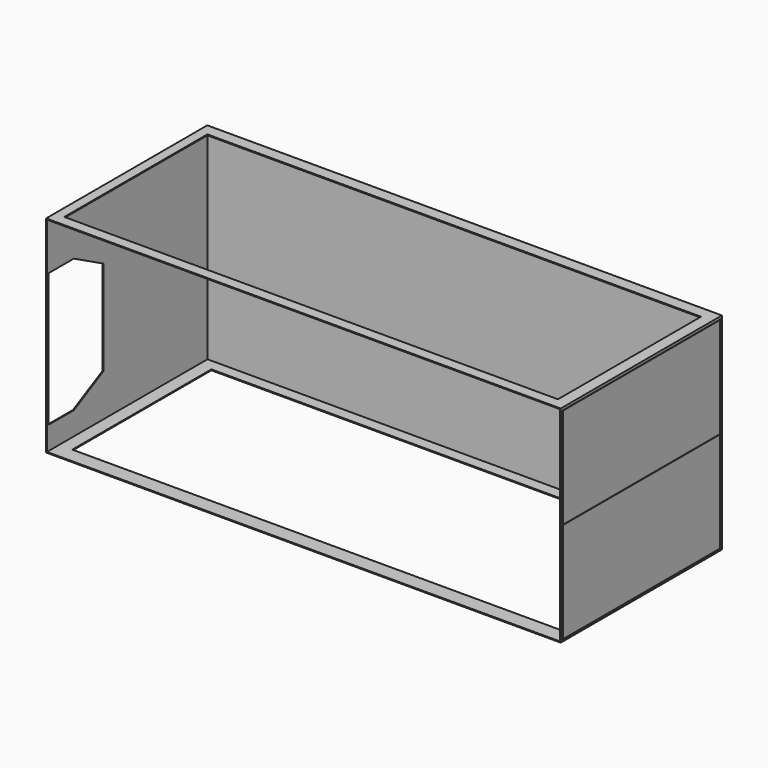
from build123d import *

# Parameters (mm, degrees)
F0_W      = 5848
F0_H      = 2343
F0_W_2    = 5828
F0_H_2    = 2323
F1_DEPTH  = 2280
F2_W      = 5848
F2_H      = 2343
F2_W_2    = 5828
F2_H_2    = 2323
F3_DEPTH  = 10
F4_W      = 5538.9823913574
F4_H      = 1975.0258177519
F5_DEPTH  = 25
F7_DEPTH  = 25
F8_W      = 2228.7018108368
F8_H      = 10
F8_W_2    = 2230
F9_DEPTH  = 5
F10_W     = 5609.335899353
F10_H     = 2031.7305922508
F11_DEPTH = 25


# Not quite as in the source:
# - a feature names something its author has since deleted; it is built from what else it names


with BuildPart() as f1:
    # F0 (on Front) → F1 (new body)
    with BuildSketch(Plane.XZ):
        Rectangle(F0_W, F0_H)
        Rectangle(F0_W_2, F0_H_2, mode=Mode.SUBTRACT)
    extrude(amount=F1_DEPTH)

    # F2 (on face) → F3 (join)
    with BuildSketch(Plane(origin=(0, 0, 0), x_dir=(-1, 0, 0), z_dir=(0, 1, 0))):
        Rectangle(F2_W, F2_H)
        Rectangle(F2_W_2, F2_H_2, mode=Mode.SUBTRACT)
        Rectangle(F2_W_2, F2_H_2)
    extrude(amount=F3_DEPTH)

    # F4 (on face) → F5 (cut)
    with BuildSketch(Plane(origin=(0, 0, -1171.5), x_dir=(1, 0, 0), z_dir=(0, 0, -1))):
        with Locations((3.7124156952, 1117.349781096)):
            Rectangle(F4_W, F4_H)
    extrude(amount=-F5_DEPTH, mode=Mode.SUBTRACT)

    # F6 (on face) → F7 (cut)
    with BuildSketch(Plane(origin=(-2924, 0, 0), x_dir=(0, -1, 0), z_dir=(-1, 0, 0))):
        Polygon((2260, -900), (2260, 616.9540286064), (1898.0355262756, 616.9540286064), (1480, 397.9138715092), (1480, -680.9598410104), (1898.03553, -900), (2053.3208847046, -900), align=None)
    extrude(amount=-F7_DEPTH, mode=Mode.SUBTRACT)

    # F8 (on face) → F9 (cut)
    with BuildSketch(Plane.YZ.offset(2924)):
        Polygon((-2248.7018108368, 1.6998175904), (-2260, 1.6998175904), (-2260, -8.3001824096), (-2250, -8.3001824096), (-2248.7018108368, -8.3001824096), (-20, -8.3001824096), (-10, -8.3001824096), (-10, 1.6998175904), (-20, 1.6998175904), align=None)
        Polygon((-20, 1136.6998175904), (-20, 1.6998175904), (-10, 1.6998175904), (-10, 1146.6998175904), (-20, 1146.6998175904), align=None)
        with Locations((-1134.3509054184, 1141.6998175904)):
            Rectangle(F8_W, F8_H)
        Polygon((-2260, 1146.6998175904), (-2260, 1.6998175904), (-2248.7018108368, 1.6998175904), (-2248.7018108368, 1136.6998175904), (-2248.7018108368, 1146.6998175904), align=None)
        Polygon((-2250, -8.3001824096), (-2260, -8.3001824096), (-2260, -1153.3001824096), (-2250, -1153.3001824096), (-2250, -1143.3001824096), align=None)
        with Locations((-1135, -1148.3001824096)):
            Rectangle(F8_W_2, F8_H)
        Polygon((-10, -1153.3001824096), (-10, -8.3001824096), (-20, -8.3001824096), (-20, -1143.3001824096), (-20, -1153.3001824096), align=None)
    extrude(amount=-F9_DEPTH, mode=Mode.SUBTRACT)

    # F10 (on face) → F11 (cut)
    with BuildSketch(Plane.XY.offset(1171.5)):
        with Locations((-10.3087425232, -1141.2568390369)):
            Rectangle(F10_W, F10_H)
    extrude(amount=-F11_DEPTH, mode=Mode.SUBTRACT)


solid = f1.part
